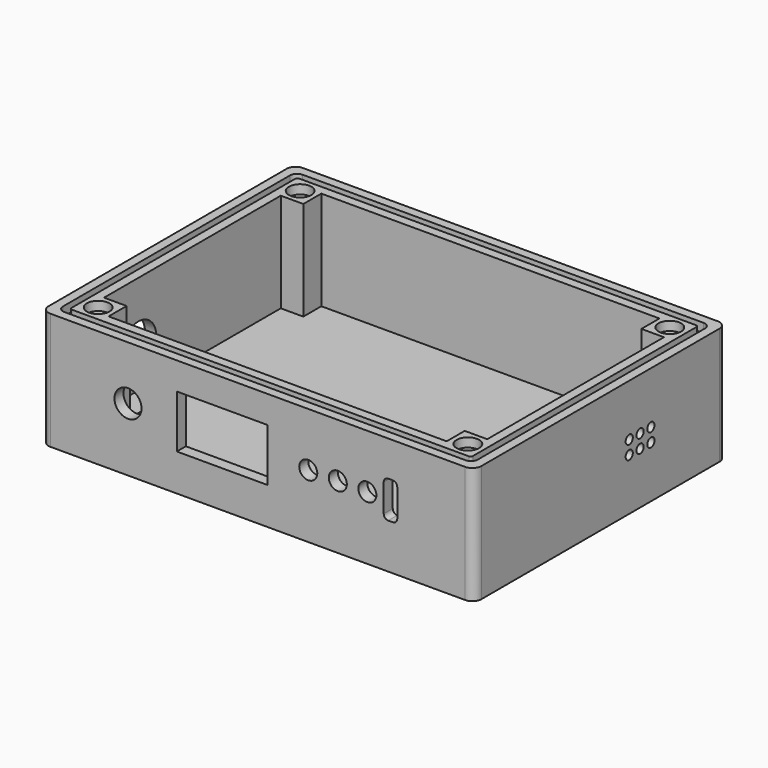
from build123d import *

# Parameters (mm, degrees)
F1_DEPTH  = 26
F3_DEPTH  = 2
F4_R      = 2.5
F5_DEPTH  = 2
F6_W      = 5
F6_H      = 49
F6_W_2    = 75
F6_H_2    = 5
F7_DEPTH  = 22
F8_R      = 1
F9_DEPTH  = 5.5
F10_R     = 11.25
F10_R_2   = 5
F11_DEPTH = 3
F12_DEPTH = 5.5
F13_W     = 20.16
F13_H     = 11.72
F13_R     = 3
F13_R_2   = 2
F14_DEPTH = 5.5
F13_W_2   = 66
F13_H_2   = 18
F13_R_3   = 1.8
F15_DEPTH = 3
F16_DEPTH = 3
F13_R_4   = 0.8
F17_DEPTH = 1.9
F18_DEPTH = 1.9
F19_DEPTH = 1.9


# Not quite as in the source:
# - a feature names something its author has since deleted; it is built from what else it names


with BuildPart() as f1:
    # F0 (on Top) → F1 (new body)
    with BuildSketch(Plane.XY):
        with BuildLine():
            Line((46, 35), (-46, 35))
            ThreePointArc((-46, 35), (-47.4142135624, 34.4142135624), (-48, 33))
            Line((-48, 33), (-48, -33))
            ThreePointArc((-48, -33), (-47.4142135624, -34.4142135624), (-46, -35))
            Line((-46, -35), (46, -35))
            ThreePointArc((46, -35), (47.4142135624, -34.4142135624), (48, -33))
            Line((48, -33), (48, 33))
            ThreePointArc((48, 33), (47.4142135624, 34.4142135624), (46, 35))
        make_face()
    extrude(amount=F1_DEPTH)

    # F2 (on face) → F3 (cut)
    with BuildSketch(Plane.XY.offset(26)):
        with BuildLine():
            Line((44.5, 33), (-44.5, 33))
            ThreePointArc((-44.5, 33), (-45.5606601718, 32.5606601718), (-46, 31.5))
            Line((-46, 31.5), (-46, -31.5))
            ThreePointArc((-46, -31.5), (-45.5606601718, -32.5606601718), (-44.5, -33))
            Line((-44.5, -33), (44.5, -33))
            ThreePointArc((44.5, -33), (45.5606601718, -32.5606601718), (46, -31.5))
            Line((46, -31.5), (46, 31.5))
            ThreePointArc((46, 31.5), (45.5606601718, 32.5606601718), (44.5, 33))
        make_face()
        with BuildLine():
            ThreePointArc((-44.5, 31), (-44.3535533906, 31.3535533906), (-44, 31.5))
            Line((-44, 31.5), (44, 31.5))
            ThreePointArc((44, 31.5), (44.3535533906, 31.3535533906), (44.5, 31))
            Line((44.5, 31), (44.5, -31))
            ThreePointArc((44.5, -31), (44.3535533906, -31.3535533906), (44, -31.5))
            Line((44, -31.5), (-44, -31.5))
            ThreePointArc((-44, -31.5), (-44.3535533906, -31.3535533906), (-44.5, -31))
            Line((-44.5, -31), (-44.5, 31))
        make_face(mode=Mode.SUBTRACT)
    extrude(amount=-F3_DEPTH, mode=Mode.SUBTRACT)

    # F4 (on face) → F5 (cut)
    with BuildSketch(Plane.XY.offset(26)):
        with Locations((-41, -28)):
            Circle(F4_R)
        with Locations((-40.9999984205, 28)):
            Circle(F4_R)
        with Locations((41, 28)):
            Circle(F4_R)
        with Locations((41, -28)):
            Circle(F4_R)
    extrude(amount=-F5_DEPTH, mode=Mode.SUBTRACT)

    # F6 (on face) → F7 (cut)
    with BuildSketch(Plane.XY.offset(26)):
        with Locations((-40, 0)):
            Rectangle(F6_W, F6_H)
        with Locations((0, -27)):
            Rectangle(F6_W_2, F6_H_2)
        Rectangle(F6_W_2, F6_H)
        with Locations((0, 27)):
            Rectangle(F6_W_2, F6_H_2)
        with Locations((40, 0)):
            Rectangle(F6_W, F6_H)
    extrude(amount=-F7_DEPTH, mode=Mode.SUBTRACT)

    # F8 (on face) → F9 (cut, through all)
    with BuildSketch(Plane.YZ.offset(48)):
        with Locations((7.9999985173, 14.5000000224)):
            Circle(F8_R)
        with Locations((7.9999985173, 11.5000000224)):
            Circle(F8_R)
        with Locations((10.9999985173, 11.5000000224)):
            Circle(F8_R)
        with Locations((10.9999985173, 14.5000000224)):
            Circle(F8_R)
        with Locations((13.9999985173, 14.5000000224)):
            Circle(F8_R)
        with Locations((13.9999985173, 11.5000000224)):
            Circle(F8_R)
    extrude(amount=-F9_DEPTH, mode=Mode.SUBTRACT)

    # F10 (on face) → F11 (cut)
    with BuildSketch(Plane(origin=(-48, 0, 0), x_dir=(0, -1, 0), z_dir=(-1, 0, 0))):
        with Locations((15, 12.5000002682)):
            Circle(F10_R)
        with Locations((15, 12.5000002682)):
            Circle(F10_R_2, mode=Mode.SUBTRACT)
    extrude(amount=-F11_DEPTH, mode=Mode.SUBTRACT)

    # F10 (on face) → F12 (cut, through all)
    with BuildSketch(Plane(origin=(-48, 0, 0), x_dir=(0, -1, 0), z_dir=(-1, 0, 0))):
        with Locations((15, 12.5000002682)):
            Circle(F10_R_2)
    extrude(amount=-F12_DEPTH, mode=Mode.SUBTRACT)

    # F13 (on face) → F14 (cut, through all)
    with BuildSketch(Plane(origin=(0, -29.5, 0), x_dir=(-1, 0, 0), z_dir=(0, 1, 0))):
        with Locations((7.8799169147, 14.0678631142)):
            Rectangle(F13_W, F13_H)
        with Locations((28.7899169147, 14.0678631142)):
            Circle(F13_R)
        with Locations((-11.2000830853, 14.0678631142)):
            Circle(F13_R_2)
        with Locations((-17.7600830853, 14.0678631142)):
            Circle(F13_R_2)
        with Locations((-24.3100830853, 14.0678631142)):
            Circle(F13_R_2)
        with BuildLine():
            ThreePointArc((-30.9400830853, 10.9678631142), (-30.6471898665, 10.260756333), (-29.9400830853, 9.9678631142))
            Line((-29.9400830853, 9.9678631142), (-28.9400830853, 9.9678631142))
            ThreePointArc((-28.9400830853, 9.9678631142), (-28.2329763041, 10.260756333), (-27.9400830853, 10.9678631142))
            Line((-27.9400830853, 10.9678631142), (-27.9400830853, 17.1678631142))
            ThreePointArc((-27.9400830853, 17.1678631142), (-28.2329763041, 17.8749698954), (-28.9400830853, 18.1678631142))
            Line((-28.9400830853, 18.1678631142), (-29.9400830853, 18.1678631142))
            ThreePointArc((-29.9400830853, 18.1678631142), (-30.6471898665, 17.8749698954), (-30.9400830853, 17.1678631142))
            Line((-30.9400830853, 17.1678631142), (-30.9400830853, 10.9678631142))
        make_face()
    extrude(amount=-F14_DEPTH, mode=Mode.SUBTRACT)

    # F13 (on face) → F15 (cut)
    with BuildSketch(Plane(origin=(0, -29.5, 0), x_dir=(-1, 0, 0), z_dir=(0, 1, 0))):
        with Locations((-0.2100830853, 14.0678631142)):
            Rectangle(F13_W_2, F13_H_2)
        with BuildLine():
            Line((-28.9400830853, 9.9678631142), (-29.9400830853, 9.9678631142))
            ThreePointArc((-29.9400830853, 9.9678631142), (-30.6471898665, 10.260756333), (-30.9400830853, 10.9678631142))
            Line((-30.9400830853, 10.9678631142), (-30.9400830853, 17.1678631142))
            ThreePointArc((-30.9400830853, 17.1678631142), (-30.6471898665, 17.8749698954), (-29.9400830853, 18.1678631142))
            Line((-29.9400830853, 18.1678631142), (-28.9400830853, 18.1678631142))
            ThreePointArc((-28.9400830853, 18.1678631142), (-28.2329763041, 17.8749698954), (-27.9400830853, 17.1678631142))
            Line((-27.9400830853, 17.1678631142), (-27.9400830853, 10.9678631142))
            ThreePointArc((-27.9400830853, 10.9678631142), (-28.2329763041, 10.260756333), (-28.9400830853, 9.9678631142))
        make_face(mode=Mode.SUBTRACT)
        with Locations((-24.3100830853, 14.0678631142)):
            Circle(F13_R_2, mode=Mode.SUBTRACT)
        with Locations((-17.7600830853, 14.0678631142)):
            Circle(F13_R_2, mode=Mode.SUBTRACT)
        with Locations((-11.2000830853, 14.0678631142)):
            Circle(F13_R_2, mode=Mode.SUBTRACT)
        with Locations((30.1299169147, 7.5678631142)):
            Circle(F13_R_3, mode=Mode.SUBTRACT)
        with Locations((7.8799169147, 14.0678631142)):
            Rectangle(F13_W, F13_H, mode=Mode.SUBTRACT)
        with Locations((28.7899169147, 14.0678631142)):
            Circle(F13_R, mode=Mode.SUBTRACT)
        with Locations((-24.0500830853, 20.5678631142)):
            Circle(F13_R_3, mode=Mode.SUBTRACT)
        with Locations((30.1299169147, 20.5678631142)):
            Circle(F13_R_3, mode=Mode.SUBTRACT)
    extrude(amount=F15_DEPTH, mode=Mode.SUBTRACT)

    # F13 (on face) → F16 (cut)
    with BuildSketch(Plane(origin=(0, -29.5, 0), x_dir=(-1, 0, 0), z_dir=(0, 1, 0))):
        with Locations((-0.2100830853, 14.0678631142)):
            Rectangle(F13_W_2, F13_H_2)
        with BuildLine():
            Line((-28.9400830853, 9.9678631142), (-29.9400830853, 9.9678631142))
            ThreePointArc((-29.9400830853, 9.9678631142), (-30.6471898665, 10.260756333), (-30.9400830853, 10.9678631142))
            Line((-30.9400830853, 10.9678631142), (-30.9400830853, 17.1678631142))
            ThreePointArc((-30.9400830853, 17.1678631142), (-30.6471898665, 17.8749698954), (-29.9400830853, 18.1678631142))
            Line((-29.9400830853, 18.1678631142), (-28.9400830853, 18.1678631142))
            ThreePointArc((-28.9400830853, 18.1678631142), (-28.2329763041, 17.8749698954), (-27.9400830853, 17.1678631142))
            Line((-27.9400830853, 17.1678631142), (-27.9400830853, 10.9678631142))
            ThreePointArc((-27.9400830853, 10.9678631142), (-28.2329763041, 10.260756333), (-28.9400830853, 9.9678631142))
        make_face(mode=Mode.SUBTRACT)
        with Locations((-24.3100830853, 14.0678631142)):
            Circle(F13_R_2, mode=Mode.SUBTRACT)
        with Locations((-17.7600830853, 14.0678631142)):
            Circle(F13_R_2, mode=Mode.SUBTRACT)
        with Locations((-11.2000830853, 14.0678631142)):
            Circle(F13_R_2, mode=Mode.SUBTRACT)
        with Locations((30.1299169147, 7.5678631142)):
            Circle(F13_R_3, mode=Mode.SUBTRACT)
        with Locations((7.8799169147, 14.0678631142)):
            Rectangle(F13_W, F13_H, mode=Mode.SUBTRACT)
        with Locations((28.7899169147, 14.0678631142)):
            Circle(F13_R, mode=Mode.SUBTRACT)
        with Locations((-24.0500830853, 20.5678631142)):
            Circle(F13_R_3, mode=Mode.SUBTRACT)
        with Locations((30.1299169147, 20.5678631142)):
            Circle(F13_R_3, mode=Mode.SUBTRACT)
    extrude(amount=-F16_DEPTH, mode=Mode.SUBTRACT)

    # F13 (on face) → F17 (join)
    with BuildSketch(Plane(origin=(0, -29.5, 0), x_dir=(-1, 0, 0), z_dir=(0, 1, 0))):
        with Locations((30.1299169147, 20.5678631142)):
            Circle(F13_R_3)
        with Locations((30.1299169147, 20.5678631142)):
            Circle(F13_R_4, mode=Mode.SUBTRACT)
    extrude(amount=F17_DEPTH)

    # F13 (on face) → F18 (join)
    with BuildSketch(Plane(origin=(0, -29.5, 0), x_dir=(-1, 0, 0), z_dir=(0, 1, 0))):
        with Locations((30.1299169147, 7.5678631142)):
            Circle(F13_R_3)
        with Locations((30.1299169147, 7.5678631142)):
            Circle(F13_R_4, mode=Mode.SUBTRACT)
    extrude(amount=F18_DEPTH)

    # F13 (on face) → F19 (join)
    with BuildSketch(Plane(origin=(0, -29.5, 0), x_dir=(-1, 0, 0), z_dir=(0, 1, 0))):
        with Locations((-24.0500830853, 20.5678631142)):
            Circle(F13_R_3)
        with Locations((-24.0500830853, 20.5678631142)):
            Circle(F13_R_4, mode=Mode.SUBTRACT)
    extrude(amount=F19_DEPTH)


solid = f1.part
